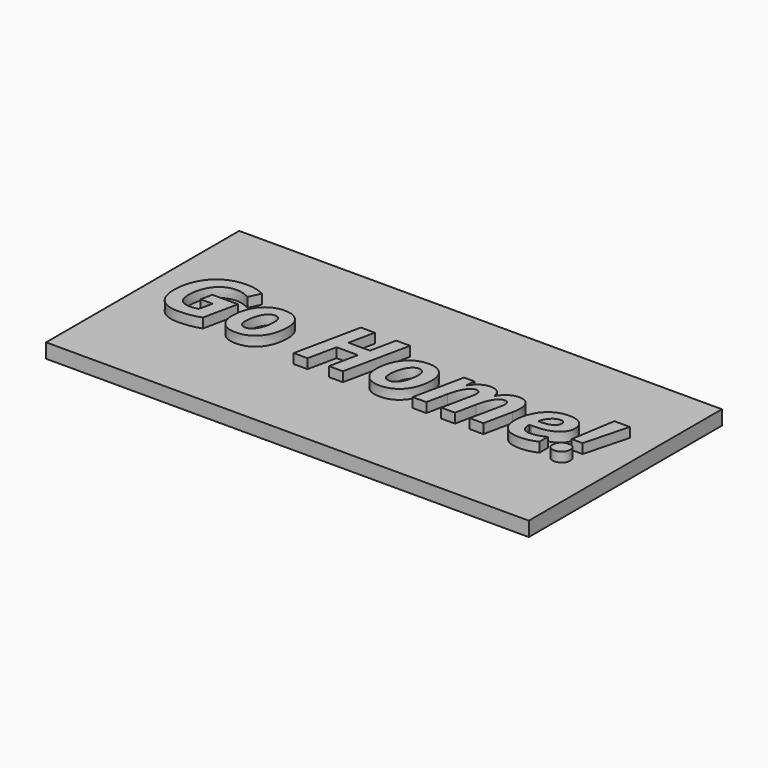
from build123d import *

# Parameters (mm, degrees)
F0_W         = 100
F0_H         = 50
F1_DEPTH     = 3
F2_TEXT_SIZE = 19.301655385
F3_DEPTH     = 2


# Not quite as in the source:
# - Text() gives the source's letters only with a copy of the font that has no kerning and outlines rounded to 1/6400 em; it was checked with that copy


with BuildPart() as f1:
    # F0 (on Top) → F1 (new body)
    with BuildSketch(Plane.XY):
        with Locations((-50, 25)):
            Rectangle(F0_W, F0_H)
    extrude(amount=F1_DEPTH)

    # F2 (on face) → F3 (join)
    with BuildSketch(Plane.XY.offset(3)):
        with Locations((-94.1088690492, 19.0733092416)):
            Text('Go Home!', F2_TEXT_SIZE, font='Open Sans', font_style=FontStyle.BOLDITALIC, text_align=(TextAlign.LEFT, TextAlign.BOTTOM))
    extrude(amount=F3_DEPTH)


solid = f1.part
